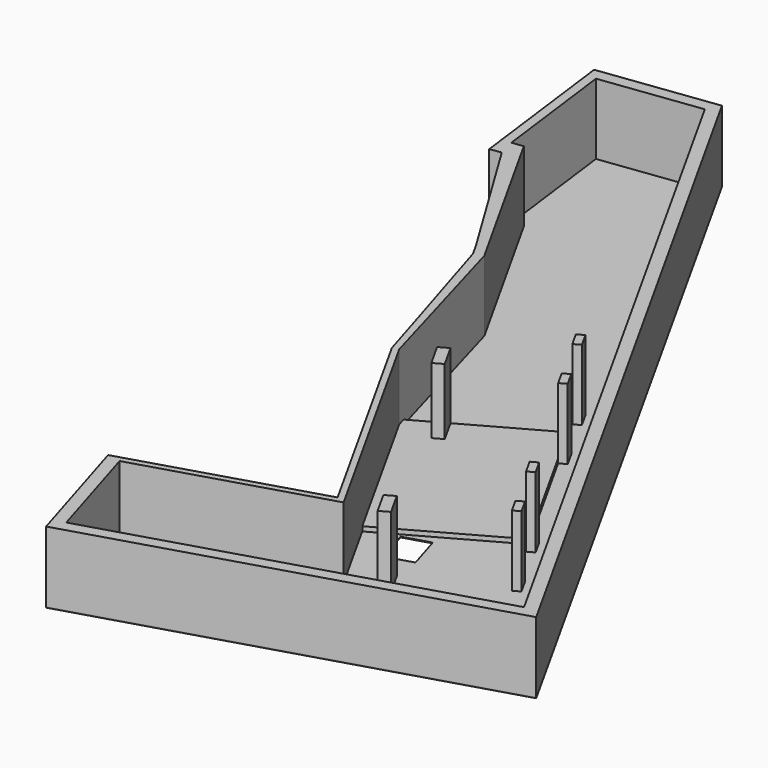
from build123d import *

# Parameters (mm, degrees)
F3_DEPTH  = 2330
F5_DEPTH  = 25
F7_DEPTH  = 2330
F9_DEPTH  = 150
F11_DEPTH = 25.001


# Not quite as in the source:
# - ends of sketch curves that miss each other by under 0.0002 mm in the source are joined


with BuildPart() as f3:
    # F2 (on Top) → F3 (new body)
    with BuildSketch(Plane.XY):
        Polygon((52902.0595629306, 50434.1230428591), (54145.32292, 46326.602018), (54431.4219269024, 46413.1983883223), (67150.915474, 50263.131268), (53075.201891, 75510.702684), (49253.5741891713, 75020.4629237414), (49304.213105, 74623.774346), (49909.660074, 69880.902321), (50281.682258, 69933.639978), (53000.597675, 65468.812402), (53225.019852, 65066.306629), (54325.972768, 61474.063518), (54760.522861, 60038.387295), (54874.022799, 59663.37285), (58991.897227, 52278.191447), (57604.002801, 51858.903346), (53909.97748, 50739.1999), align=None)
        Polygon((54412.25928, 46825.31334), (53342.81403, 50358.57026), (59287.509616, 52158.706562), (55070.827017, 59721.094989), (53523.858293, 65159.740021), (50504.389213421, 70561.8996273451), (50131.257661, 70514.151722), (49601.798244, 74661.762303), (52857.629236, 75079.514646), (66559.719817, 50502.109853), align=None, mode=Mode.SUBTRACT)
    extrude(amount=F3_DEPTH)


with BuildPart() as f5:
    # F4 (on Top) → F5 (new body)
    with BuildSketch(Plane.XY):
        Polygon((54760.522861, 60038.387295), (54874.022799, 59663.37285), (58991.897227, 52278.191447), (57604.002801, 51858.903346), (53909.97748, 50739.1999), (52902.0595629306, 50434.1230428591), (54145.32292, 46326.602018), (67150.915474, 50263.131268), (53075.201891, 75510.702684), (49253.5741891713, 75020.4629237414), (49304.213105, 74623.774346), (49909.660074, 69880.902321), (50281.682258, 69933.639978), (53000.597675, 65468.812402), (53225.019852, 65066.306629), (54325.972768, 61474.063518), align=None)
    extrude(amount=-F5_DEPTH)

    # F6 (on Top) → F7 (join)
    with BuildSketch(Plane.XY):
        Polygon((63167.175561, 54636.370609), (62899.326908, 55116.742443), (62680.976074, 54994.993056), (62948.824727, 54514.621222), align=None)
        Polygon((61606.57177, 56922.149305), (61874.420423, 56441.777471), (62092.771256, 56563.526859), (61824.922604, 57043.898693), align=None)
        Polygon((60131.75578, 53293.714353), (59826.064613, 53123.26521), (60264.362406, 52337.202212), (60570.053573, 52507.651355), align=None)
        Polygon((56498.652366, 59810.307311), (56060.354571, 60596.370312), (55754.663404, 60425.921169), (56192.961199, 59639.858168), align=None)
        Polygon((59393.320264, 61405.457583), (59174.969431, 61283.708196), (59442.818085, 60803.336359), (59661.168918, 60925.085747), align=None)
        Polygon((58586.764842, 62852.241589), (58318.916189, 63332.613423), (58100.565355, 63210.864035), (58368.414008, 62730.492201), align=None)
    extrude(amount=F7_DEPTH)

    # F10 (on face) → F11 (cut, through all)
    with BuildSketch(Plane.XY):
        Polygon((59168.735458, 53933.31513), (60028.231633, 54193.415485), (59680.654869, 55341.975624), (58821.158694, 55081.875269), align=None)
    extrude(amount=-F11_DEPTH, mode=Mode.SUBTRACT)


with BuildPart() as f9:
    # F8 (on Top) → F9 (new body)
    with BuildSketch(Plane.XY):
        Polygon((58728.797232615, 62084.088870835), (56060.354571, 60596.370312), (56498.652366, 59810.307311), (56192.961199, 59639.858168), (55754.663404, 60425.921169), (54991.3996931603, 60000.3359416475), (55070.827017, 59721.094989), (55102.8168784927, 59663.7229310719), (57874.844064254, 54692.2445670372), (58565.3824039826, 55077.2791403316), (61670.1839855803, 56808.2778988538), align=None)
    extrude(amount=F9_DEPTH)


solid = Compound([f3.part, f5.part, f9.part])
